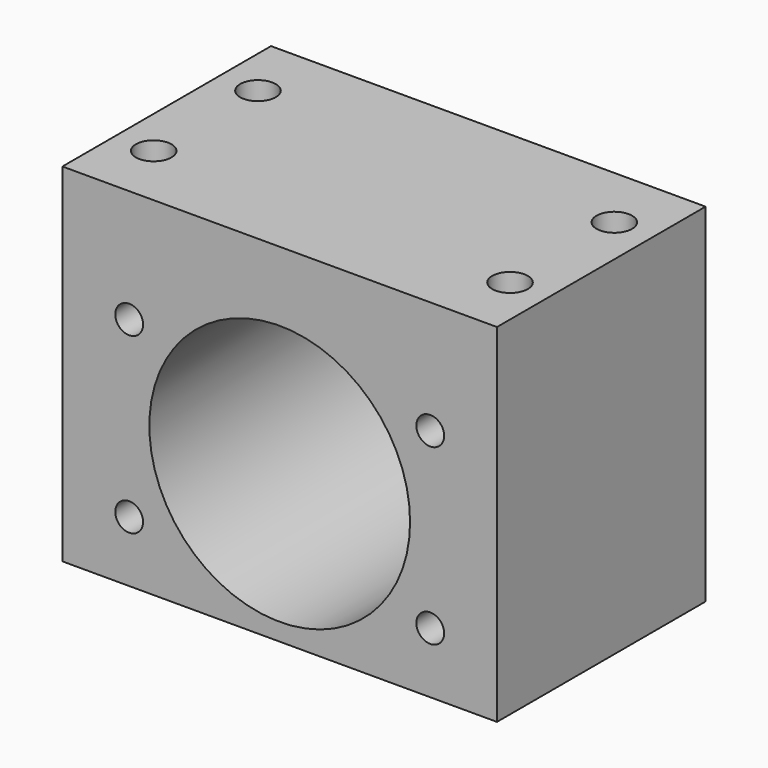
from build123d import *

# Parameters (mm, degrees)
F0_W     = 50
F0_H     = 40
F1_DEPTH = 30
F2_R     = 15
F3_DEPTH = 30.001
F4_D     = 3.2
F6_D     = 4.1


# Not quite as in the source:
# - a feature names something its author has since deleted; it is built from what else it names


with BuildPart() as f1:
    # F0 (on Front) → F1 (new body)
    with BuildSketch(Plane.XZ):
        with Locations((3.412880823, -1.3936108311)):
            Rectangle(F0_W, F0_H)
    extrude(amount=F1_DEPTH)

    # F2 (on face) → F3 (cut, through all)
    with BuildSketch(Plane.XZ.offset(30)):
        with Locations((3.412880823, -4.3936108311)):
            Circle(F2_R)
    extrude(amount=-F3_DEPTH, mode=Mode.SUBTRACT)

    # F4 (through all)
    with Locations(Plane.XZ.offset(30)):
        with Locations((-13.9076272527, -14.3936108311), (-13.9076272527, 5.6063891689), (20.7333888987, 5.6063891689), (20.7333888987, -14.3936108311)):
            Hole(F4_D / 2)

    # F6 (through all)
    with Locations(Plane.XY.offset(18.6063891689)):
        with Locations((23.912880823, -22.5), (23.912880823, -7.5), (-17.087119177, -7.5), (-17.087119177, -22.5)):
            Hole(F6_D / 2)


solid = f1.part
